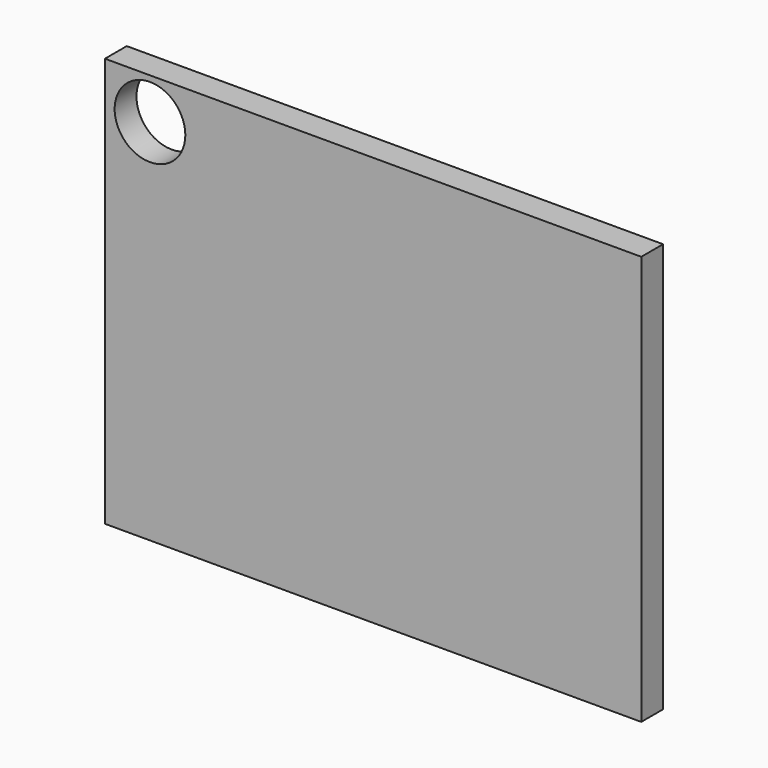
from build123d import *

# Parameters (mm, degrees)
F0_W         = 98.3252599835
F0_H         = 75.0684142113
F0_R         = 6.477687652
F1_DEPTH     = 5
F2_TEXT_SIZE = 13.7186428118
F3_DEPTH     = 5
F4_DEPTH     = 3
F5_DEPTH     = 5


# Not quite as in the source:
# - Text() gives the source's letters only with a copy of the font that has no kerning and outlines rounded to 1/6400 em; it was checked with that copy


with BuildPart() as f1:
    # F0 (on Front) → F1 (new body)
    with BuildSketch(Plane.XZ):
        with Locations((-49.1626299918, 37.5342071056)):
            Rectangle(F0_W, F0_H)
        with Locations((-90.0641456246, 67.5256624818)):
            Circle(F0_R, mode=Mode.SUBTRACT)
    extrude(amount=F1_DEPTH)

    # F2 (on Front) → F3 (join)
    with BuildSketch(Plane.XZ):
        with Locations((-96.1701869965, 28.1955543905)):
            Text('Nic', F2_TEXT_SIZE, font='Open Sans', font_style=FontStyle.ITALIC, text_align=(TextAlign.LEFT, TextAlign.BOTTOM))
    extrude(amount=F3_DEPTH)

    # F2 (on Front) → F4 (join)
    with BuildSketch(Plane.XZ):
        with Locations((-96.1701869965, 28.1955543905)):
            Text('Nic', F2_TEXT_SIZE, font='Open Sans', font_style=FontStyle.ITALIC, text_align=(TextAlign.LEFT, TextAlign.BOTTOM))
    extrude(amount=F4_DEPTH)

    # F2 (on Front) → F5 (join)
    with BuildSketch(Plane.XZ):
        with Locations((-96.1701869965, 28.1955543905)):
            Text('Nic', F2_TEXT_SIZE, font='Open Sans', font_style=FontStyle.ITALIC, text_align=(TextAlign.LEFT, TextAlign.BOTTOM))
    extrude(amount=F5_DEPTH)


solid = f1.part
